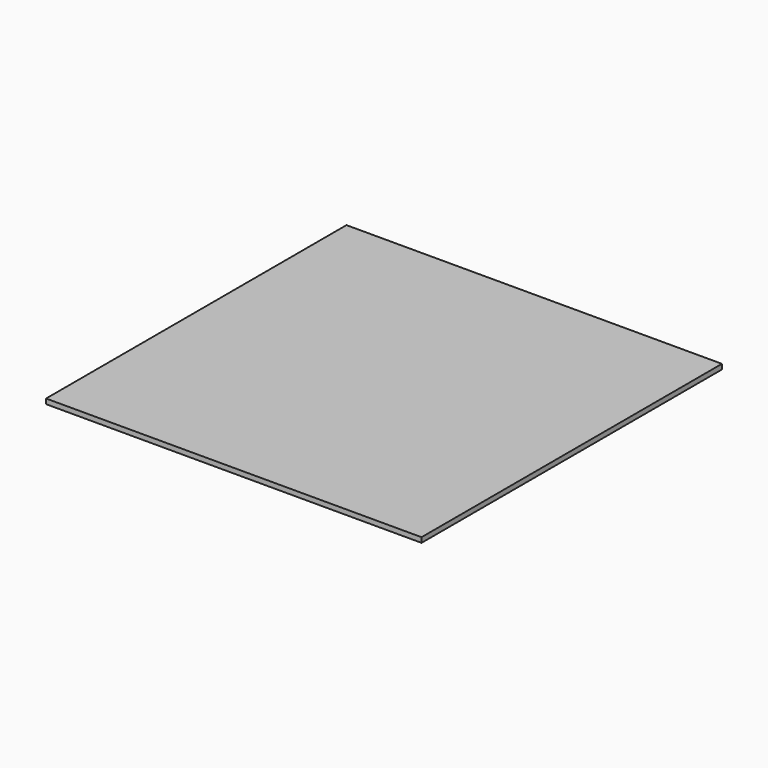
from build123d import *

# Parameters (mm, degrees)
F0_W     = 150
F0_H     = 150
F1_DEPTH = 2


# Not quite as in the source:
# - the program builds the solid bodies; features that only make, move or delete a surface that nothing else refers to are left out


with BuildPart() as f1:
    # F0 (on Top) → F1 (new body)
    with BuildSketch(Plane.XY):
        Rectangle(F0_W, F0_H)
    extrude(amount=F1_DEPTH)


solid = f1.part
